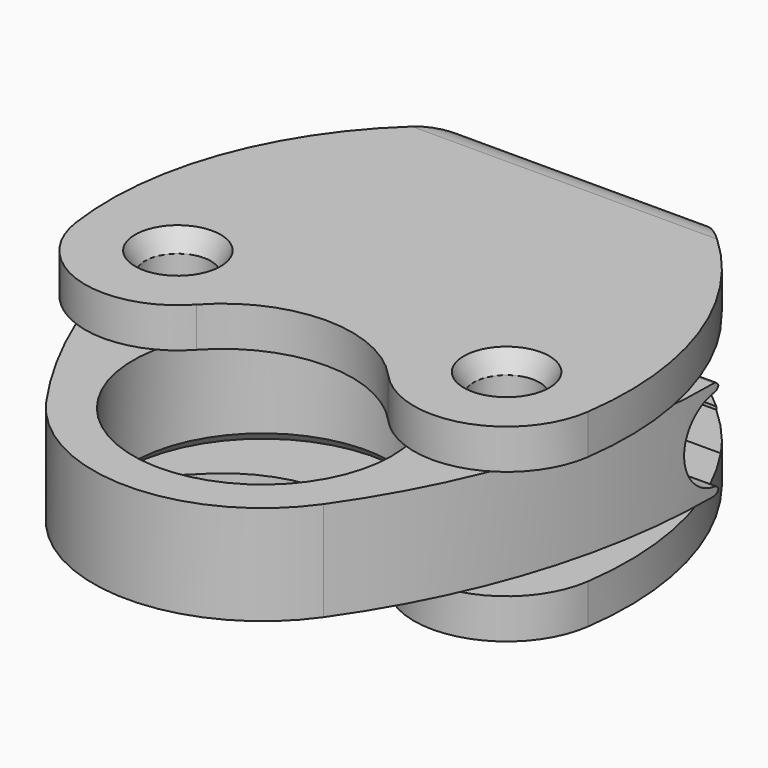
from build123d import *

# Parameters (mm, degrees)
F0_R        = 6.5
F0_R_2      = 1.65
F1_DEPTH    = 2.5
F2_R        = 2.1
F3_DEPTH    = 19.8
F2_W        = 8.2
F2_H        = 6
F4_DEPTH    = 6
F5_T1_DEPTH = 7.9058808998
F5_T3_DEPTH = 7.9058808998
F5_T5_DEPTH = 8
F5_T7_DEPTH = 8
F6_SIZE     = 0.5
F7_SIZE2    = 0.5
F7_SIZE     = 1
F7_2_SIZE2  = 0.5
F7_2_SIZE   = 1
F8_W        = 10
F8_H        = 11.7595842183
F9_DEPTH    = 4.75
F10_START   = 2.75
F8_R        = 1.65
F10_DEPTH   = 2
F11_START   = -2.75
F11_DEPTH   = 2
F12_DEPTH   = 12.5
F13_W       = 3
F13_H       = 5.8
F14_DEPTH   = 12.5
F16_D       = 3.2
F16_DEPTH   = 7.5
F16_TIP     = 0.9613769904
F17_SIZE    = 0.5
F18_R       = 2
F19_SIZE2   = 0.5
F19_SIZE    = 1
F19_2_SIZE2 = 0.5
F19_2_SIZE  = 1
F19_3_SIZE2 = 0.5
F19_3_SIZE  = 1
F19_4_SIZE2 = 0.5
F19_4_SIZE  = 1
F20_SIZE2   = 0.5
F20_SIZE    = 1


# Not quite as in the source:
# - a fillet or chamfer that OpenCascade refuses, or shapes differently, is made with other operations: its cross-section is extruded or revolved along the edge and cut away or added


with BuildPart() as f1:
    # F0 (on Top) → F1 (new body, symmetric)
    with BuildSketch(Plane.XY):
        with BuildLine():
            ThreePointArc((-12.5, 13), (-11.1303999816, 3.6282915772), (-6.9620872127, -4.8764066323))
            ThreePointArc((-6.9620872127, -4.8764066323), (0, -8.5), (6.9620872127, -4.8764066323))
            ThreePointArc((6.9620872127, -4.8764066323), (11.1303999816, 3.6282915772), (12.5, 13))
            Line((12.5, 13), (-12.5, 13))
        make_face()
        Circle(F0_R, mode=Mode.SUBTRACT)
        with Locations((-8.2536355626, 5)):
            Circle(F0_R_2, mode=Mode.SUBTRACT)
        with Locations((8.2536355626, 5)):
            Circle(F0_R_2, mode=Mode.SUBTRACT)
    extrude(amount=F1_DEPTH, both=True)

    # F2 (on Right) → F3 (cut, symmetric)
    with BuildSketch(Plane.YZ):
        with Locations((13, 0)):
            Circle(F2_R)
    extrude(amount=F3_DEPTH, both=True, mode=Mode.SUBTRACT)

    # F2 (on Right) → F4 (cut, symmetric)
    with BuildSketch(Plane.YZ):
        with Locations((13, 0)):
            Rectangle(F2_W, F2_H)
        with Locations((13, 0)):
            Circle(F2_R, mode=Mode.SUBTRACT)
    extrude(amount=F4_DEPTH, both=True, mode=Mode.SUBTRACT)

    # F5: fillet of radius 0.3 on 8 edges, made by hand

    # F5_s2 → F5_t1 (cut)
    with BuildSketch(Plane.YZ.offset(5.2970595501)):
        with BuildLine():
            ThreePointArc((13, 2.38117618), (12.925, 2.1827448316), (12.7375, 2.0835291575))
            ThreePointArc((12.7375, 2.0835291575), (12.8684918837, 2.0958782444), (13, 2.1))
            Line((13, 2.1), (13, 2.38117618))
        make_face()
        with BuildLine():
            ThreePointArc((12.7375, -2.0835291575), (12.925, -2.1827448316), (13, -2.38117618))
            Line((13, -2.38117618), (13, -2.1))
            ThreePointArc((13, -2.1), (12.8684918837, -2.0958782444), (12.7375, -2.0835291575))
        make_face()
    extrude(amount=F5_T1_DEPTH, mode=Mode.SUBTRACT)

    # F5_s4 → F5_t3 (cut)
    with BuildSketch(Plane.YZ.offset(-13.2029404499)):
        with BuildLine():
            ThreePointArc((13, 2.38117618), (12.925, 2.1827448316), (12.7375, 2.0835291575))
            ThreePointArc((12.7375, 2.0835291575), (12.8684918837, 2.0958782444), (13, 2.1))
            Line((13, 2.1), (13, 2.38117618))
        make_face()
        with BuildLine():
            ThreePointArc((13, -2.38117618), (12.925, -2.1827448316), (12.7375, -2.0835291575))
            ThreePointArc((12.7375, -2.0835291575), (12.8684918837, -2.0958782444), (13, -2.1))
            Line((13, -2.1), (13, -2.38117618))
        make_face()
    extrude(amount=F5_T3_DEPTH, mode=Mode.SUBTRACT)

    # F5_s6 → F5_t5 (cut)
    with BuildSketch(Plane.YZ.offset(-13.25)):
        with BuildLine():
            ThreePointArc((12.7, 2.5), (12.9121320344, 2.4121320344), (13, 2.2))
            Line((13, 2.2), (13, 2.5))
            Line((13, 2.5), (12.7, 2.5))
        make_face()
        with BuildLine():
            ThreePointArc((12.7, -2.5), (12.9121320344, -2.4121320344), (13, -2.2))
            Line((13, -2.2), (13, -2.5))
            Line((13, -2.5), (12.7, -2.5))
        make_face()
    extrude(amount=F5_T5_DEPTH, mode=Mode.SUBTRACT)

    # F5_s8 → F5_t7 (cut)
    with BuildSketch(Plane.YZ.offset(5.25)):
        with BuildLine():
            ThreePointArc((12.7, 2.5), (12.9121320344, 2.4121320344), (13, 2.2))
            Line((13, 2.2), (13, 2.5))
            Line((13, 2.5), (12.7, 2.5))
        make_face()
        with BuildLine():
            ThreePointArc((13, -2.2), (12.9121320344, -2.4121320344), (12.7, -2.5))
            Line((12.7, -2.5), (13, -2.5))
            Line((13, -2.5), (13, -2.2))
        make_face()
    extrude(amount=F5_T7_DEPTH, mode=Mode.SUBTRACT)

    # F6
    f6_edges = [f1.edges().sort_by_distance(p)[0] for p in [
        (-6.5, 0, -2.5),
    ]]
    chamfer(f6_edges, length=F6_SIZE)

    # F7
    f7_edges = [f1.edges().sort_by_distance(p)[0] for p in [
        (-9.903636, 5, 2.5),
    ]]
    f7_side = f1.faces().sort_by_distance((-9.903636, 5, 0))[0]
    chamfer(f7_edges, length=F7_SIZE, length2=F7_SIZE2, reference=f7_side)

    # F7#2
    f7_2_edges = [f1.edges().sort_by_distance(p)[0] for p in [
        (6.603636, 5, 2.5),
    ]]
    f7_2_side = f1.faces().sort_by_distance((6.603636, 5, 0))[0]
    chamfer(f7_2_edges, length=F7_2_SIZE, length2=F7_2_SIZE2, reference=f7_2_side)


with BuildPart() as f9:
    # F8 (on Top) → F9 (new body, symmetric)
    with BuildSketch(Plane.XY):
        with Locations((0, 15.0797921091)):
            Rectangle(F8_W, F8_H)
    extrude(amount=F9_DEPTH, both=True)

    # F8 (on Top) → F10 (join)
    with BuildSketch(Plane.XY.offset(F10_START)):
        with BuildLine():
            Line((5, 20.9595842183), (5, 9.2))
            Line((5, 9.2), (-5, 9.2))
            Line((-5, 9.2), (-5, 20.9595842183))
            ThreePointArc((-5, 20.9595842183), (-11.4247335497, 13.830813762), (-12.8567829642, 4.3415670122))
            ThreePointArc((-12.8567829642, 4.3415670122), (-9.6188596548, 0.5549282145), (-4.8136495699, 1.8712628154))
            ThreePointArc((-4.8136495699, 1.8712628154), (0, 4), (4.8136495699, 1.8712628154))
            ThreePointArc((4.8136495699, 1.8712628154), (9.6188596548, 0.5549282145), (12.8567829642, 4.3415670122))
            ThreePointArc((12.8567829642, 4.3415670122), (11.4247335497, 13.830813762), (5, 20.9595842183))
        make_face()
        with Locations((-8.2536355626, 5)):
            Circle(F8_R, mode=Mode.SUBTRACT)
        with Locations((8.2536355626, 5)):
            Circle(F8_R, mode=Mode.SUBTRACT)
    extrude(amount=F10_DEPTH)

    # F8 (on Top) → F11 (join)
    with BuildSketch(Plane.XY.offset(F11_START)):
        with BuildLine():
            Line((5, 20.9595842183), (5, 9.2))
            Line((5, 9.2), (-5, 9.2))
            Line((-5, 9.2), (-5, 20.9595842183))
            ThreePointArc((-5, 20.9595842183), (-11.4247335497, 13.830813762), (-12.8567829642, 4.3415670122))
            ThreePointArc((-12.8567829642, 4.3415670122), (-9.6188596548, 0.5549282145), (-4.8136495699, 1.8712628154))
            ThreePointArc((-4.8136495699, 1.8712628154), (0, 4), (4.8136495699, 1.8712628154))
            ThreePointArc((4.8136495699, 1.8712628154), (9.6188596548, 0.5549282145), (12.8567829642, 4.3415670122))
            ThreePointArc((12.8567829642, 4.3415670122), (11.4247335497, 13.830813762), (5, 20.9595842183))
        make_face()
        with Locations((-8.2536355626, 5)):
            Circle(F8_R, mode=Mode.SUBTRACT)
        with Locations((8.2536355626, 5)):
            Circle(F8_R, mode=Mode.SUBTRACT)
    extrude(amount=-F11_DEPTH)

    # F2 (on Right) → F12 (cut, symmetric)
    with BuildSketch(Plane.YZ):
        with Locations((13, 0)):
            Circle(F2_R)
    extrude(amount=F12_DEPTH, both=True, mode=Mode.SUBTRACT)

    # F13 (on Right) → F14 (cut, symmetric)
    with BuildSketch(Plane.YZ):
        with Locations((17.6, 0)):
            Rectangle(F13_W, F13_H)
    extrude(amount=F14_DEPTH, both=True, mode=Mode.SUBTRACT)

    # F16
    with Locations(Plane(origin=(0, 20.9595842183, 0), x_dir=(-1, 0, 0), z_dir=(0, 1, 0))):
        with Locations((0, 0)):
            Hole(F16_D / 2, depth=F16_DEPTH)
            with Locations((0, 0, -(F16_DEPTH + F16_TIP / 2))):  # 118° drill point
                Cone(0, F16_D / 2, F16_TIP, mode=Mode.SUBTRACT)

    # F17
    f17_edges = [f9.edges().sort_by_distance(p)[0] for p in [
        (-5, 16.1, 0),
        (-5, 19.1, 0),
    ]]
    chamfer(f17_edges, length=F17_SIZE)

    # F18
    f18_edges = [f9.edges().sort_by_distance(p)[0] for p in [
        (0, 20.959584, -4.75),
        (0, 20.959584, 4.75),
    ]]
    fillet(f18_edges, radius=F18_R)

    # F19
    f19_edges = [f9.edges().sort_by_distance(p)[0] for p in [
        (-9.903636, 5, -2.75),
    ]]
    f19_side = f9.faces().sort_by_distance((-9.903636, 5, -3.75))[0]
    chamfer(f19_edges, length=F19_SIZE, length2=F19_SIZE2, reference=f19_side)

    # F19#2
    f19_2_edges = [f9.edges().sort_by_distance(p)[0] for p in [
        (6.603636, 5, -2.75),
    ]]
    f19_2_side = f9.faces().sort_by_distance((6.603636, 5, -3.75))[0]
    chamfer(f19_2_edges, length=F19_2_SIZE, length2=F19_2_SIZE2, reference=f19_2_side)

    # F19#3
    f19_3_edges = [f9.edges().sort_by_distance(p)[0] for p in [
        (-9.903636, 5, 4.75),
    ]]
    f19_3_side = f9.faces().sort_by_distance((-9.903636, 5, 3.75))[0]
    chamfer(f19_3_edges, length=F19_3_SIZE, length2=F19_3_SIZE2, reference=f19_3_side)

    # F19#4
    f19_4_edges = [f9.edges().sort_by_distance(p)[0] for p in [
        (6.603636, 5, 4.75),
    ]]
    f19_4_side = f9.faces().sort_by_distance((6.603636, 5, 3.75))[0]
    chamfer(f19_4_edges, length=F19_4_SIZE, length2=F19_4_SIZE2, reference=f19_4_side)

    # F20
    f20_edges = [f9.edges().sort_by_distance(p)[0] for p in [
        (-5, 10.9, 0),
    ]]
    f20_side = f9.faces().sort_by_distance((0, 10.9, 0))[0]
    chamfer(f20_edges, length=F20_SIZE, length2=F20_SIZE2, reference=f20_side)


solid = Compound([f1.part, f9.part])
